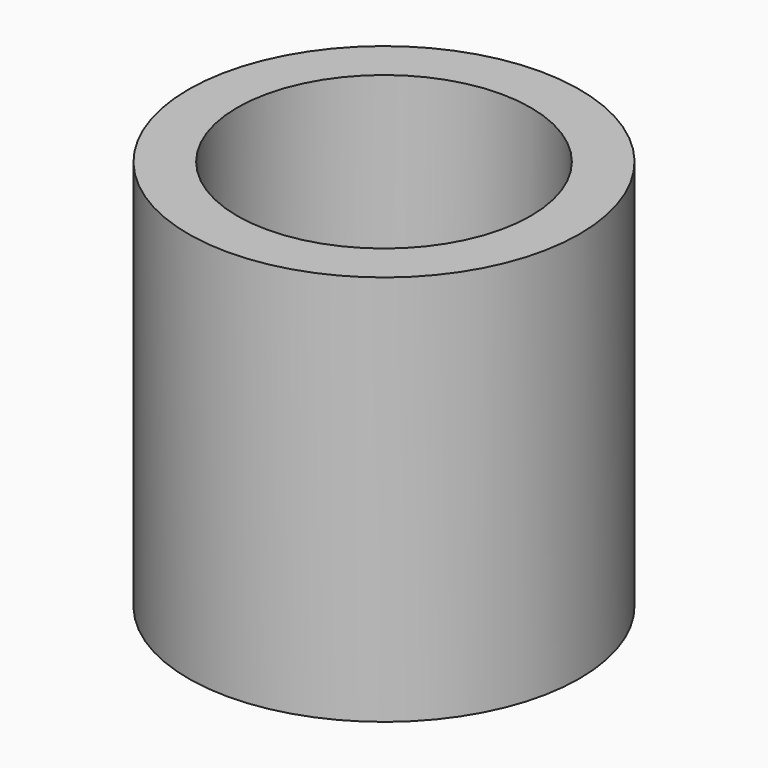
from build123d import *

# Parameters (mm, degrees)
F0_R     = 25.4
F0_R_2   = 19.05
F2_DEPTH = 50.8


# Not quite as in the source:
# - the program builds the solid bodies; features that only make, move or delete a surface that nothing else refers to are left out


with BuildPart() as f2:
    # F0 (on Top) → F2 (new body)
    with BuildSketch(Plane.XY):
        with Locations((0.0052079558, -0.1154523343)):
            Circle(F0_R)
        with Locations((0.0052079558, -0.1154523343)):
            Circle(F0_R_2, mode=Mode.SUBTRACT)
    extrude(amount=F2_DEPTH)


solid = f2.part
